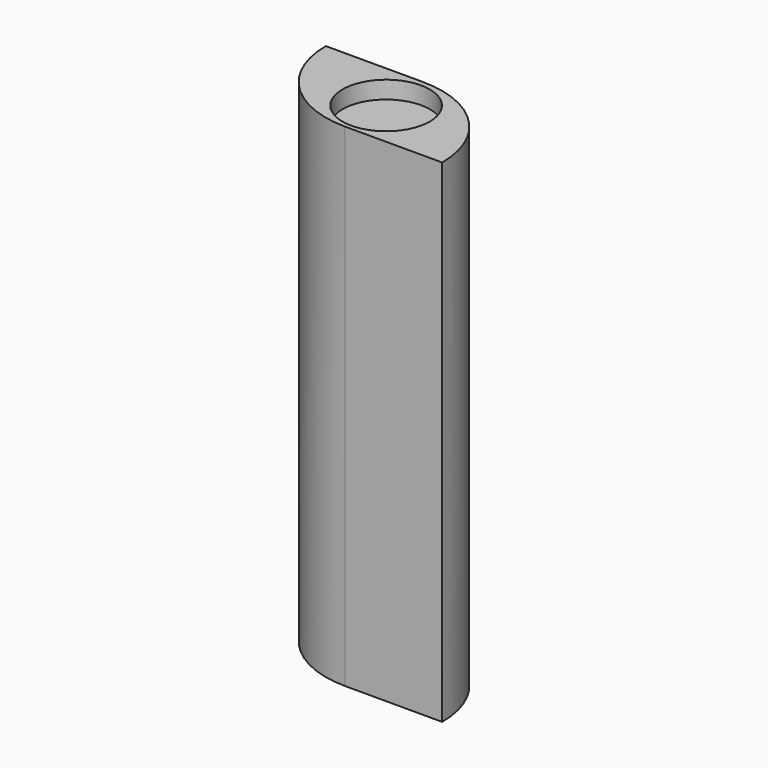
from build123d import *

# Parameters (mm, degrees)
F0_W     = 10
F0_H     = 25.4
F1_DEPTH = 5
F2_R     = 4.99999
F3_R     = 2.25
F4_DEPTH = 0.9
F5_R     = 2.25
F6_DEPTH = 0.9


# Not quite as in the source:
# - a fillet or chamfer is up to 0.001 mm smaller than in the source, because OpenCascade refuses the exact size


with BuildPart() as f1:
    # F0 (on Front) → F1 (new body)
    with BuildSketch(Plane.XZ):
        with Locations((-3.6362301892, -0.5979733542)):
            Rectangle(F0_W, F0_H)
    extrude(amount=F1_DEPTH)

    # F2 (radius 5 in the source; OpenCascade refuses exactly that, so slightly less here)
    f2_edges = [f1.edges().sort_by_distance(p)[0] for p in [
        (1.36377, 0, -0.597973),
        (-8.63623, -5, -0.597973),
    ]]
    fillet(f2_edges, radius=F2_R)

    # F3 (on face) → F4 (cut)
    with BuildSketch(Plane.XY.offset(12.1020266458)):
        with Locations((-3.5037611703, -2.5272680031)):
            Circle(F3_R)
    extrude(amount=-F4_DEPTH, mode=Mode.SUBTRACT)

    # F5 (on face) → F6 (cut)
    with BuildSketch(Plane(origin=(0, 0, -13.2979733542), x_dir=(1, 0, 0), z_dir=(0, 0, -1))):
        with Locations((-3.5220479187, 2.6191056776)):
            Circle(F5_R)
    extrude(amount=-F6_DEPTH, mode=Mode.SUBTRACT)


solid = f1.part
